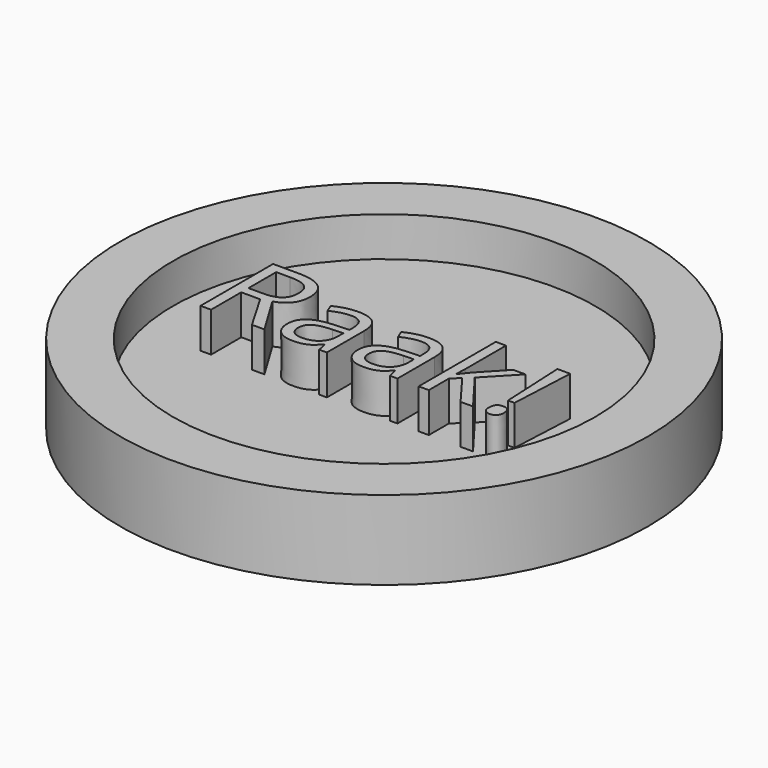
from build123d import *

# Parameters (mm, degrees)
F0_R         = 10
F0_R_2       = 8
F0_TEXT_SIZE = 4.8089487892
F1_DEPTH     = 3
F2_DEPTH     = 1.5


# Not quite as in the source:
# - Text() gives the source's letters only with a copy of the font that has no kerning and outlines rounded to 1/6400 em; it was checked with that copy


with BuildPart() as f1:
    # F0 (on Top) → F1 (new body)
    with BuildSketch(Plane.XY):
        with Locations((-7.6372292832, -17.8669122979)):
            Circle(F0_R)
        with Locations((-7.6372292832, -17.8669122979)):
            Circle(F0_R_2, mode=Mode.SUBTRACT)
        with Locations((-13.6769684032, -19.598133862)):
            Text('Raak!', F0_TEXT_SIZE, font='Open Sans', text_align=(TextAlign.LEFT, TextAlign.BOTTOM))
    extrude(amount=F1_DEPTH)

    # F0 (on Top) → F2 (join)
    with BuildSketch(Plane.XY):
        with Locations((-7.6372292832, -17.8669122979)):
            Circle(F0_R_2)
        with BuildLine():
            Line((-12.0892639045, -18.1704771902), (-12.8060978334, -18.1704771902))
            Line((-12.8060978334, -18.1704771902), (-12.8060978334, -19.598133862))
            Line((-12.8060978334, -19.598133862), (-13.2050903032, -19.598133862))
            Line((-13.2050903032, -19.598133862), (-13.2050903032, -16.1649952655))
            Line((-13.2050903032, -16.1649952655), (-12.2635882981, -16.1649952655))
            add(Edge.make_bspline(
                [(-12.2635882981, -16.1649952655), (-11.6316623713, -16.1649952655), (-11.3299759746, -16.4069455014)],
                knots=[0, 0, 0, 1, 1, 1], degree=2))
            add(Edge.make_bspline(
                [(-11.3299759746, -16.4069455014), (-11.0282895779, -16.6488957374), (-11.0282895779, -17.135050404)],
                knots=[0, 0, 0, 1, 1, 1], degree=2))
            add(Edge.make_bspline(
                [(-11.0282895779, -17.135050404), (-11.0282895779, -17.815817217), (-11.7188245681, -18.0555132582)],
                knots=[0, 0, 0, 1, 1, 1], degree=2))
            Line((-11.7188245681, -18.0555132582), (-10.7863393419, -19.598133862))
            Line((-10.7863393419, -19.598133862), (-11.2582174418, -19.598133862))
            Line((-11.2582174418, -19.598133862), (-12.0892639045, -18.1704771902))
        make_face(mode=Mode.SUBTRACT)
        with BuildLine():
            Line((-8.4194348597, -19.598133862), (-8.7087231853, -19.598133862))
            Line((-8.7087231853, -19.598133862), (-8.7861172049, -19.2314515168))
            Line((-8.7861172049, -19.2314515168), (-8.8049021611, -19.2314515168))
            add(Edge.make_bspline(
                [(-8.8049021611, -19.2314515168), (-8.9972601127, -19.4734017528), (-9.1884909669, -19.5594368522)],
                knots=[0, 0, 0, 1, 1, 1], degree=2))
            add(Edge.make_bspline(
                [(-9.1884909669, -19.5594368522), (-9.3797218211, -19.6454719517), (-9.6667559519, -19.6454719517)],
                knots=[0, 0, 0, 1, 1, 1], degree=2))
            add(Edge.make_bspline(
                [(-9.6667559519, -19.6454719517), (-10.0492176603, -19.6454719517), (-10.2663717541, -19.4478542124)],
                knots=[0, 0, 0, 1, 1, 1], degree=2))
            add(Edge.make_bspline(
                [(-10.2663717541, -19.4478542124), (-10.4835258478, -19.250236473), (-10.4835258478, -18.8865597209)],
                knots=[0, 0, 0, 1, 1, 1], degree=2))
            add(Edge.make_bspline(
                [(-10.4835258478, -18.8865597209), (-10.4835258478, -18.1073597374), (-9.2369561539, -18.0697898249)],
                knots=[0, 0, 0, 1, 1, 1], degree=2))
            Line((-9.2369561539, -18.0697898249), (-8.8003937716, -18.0555132582))
            Line((-8.8003937716, -18.0555132582), (-8.8003937716, -17.8954654313))
            add(Edge.make_bspline(
                [(-8.8003937716, -17.8954654313), (-8.8003937716, -17.5926519373), (-8.9303856686, -17.4483834736)],
                knots=[0, 0, 0, 1, 1, 1], degree=2))
            add(Edge.make_bspline(
                [(-8.9303856686, -17.4483834736), (-9.0603775655, -17.3041150099), (-9.3474116964, -17.3041150099)],
                knots=[0, 0, 0, 1, 1, 1], degree=2))
            add(Edge.make_bspline(
                [(-9.3474116964, -17.3041150099), (-9.6690101467, -17.3041150099), (-10.0747652007, -17.500981351)],
                knots=[0, 0, 0, 1, 1, 1], degree=2))
            Line((-10.0747652007, -17.500981351), (-10.1949889205, -17.2026762464))
            add(Edge.make_bspline(
                [(-10.1949889205, -17.2026762464), (-10.0048851637, -17.0997346864), (-9.7783385918, -17.041125623)],
                knots=[0, 0, 0, 1, 1, 1], degree=2))
            add(Edge.make_bspline(
                [(-9.7783385918, -17.041125623), (-9.5517920199, -16.9825165596), (-9.3233669524, -16.9825165596)],
                knots=[0, 0, 0, 1, 1, 1], degree=2))
            add(Edge.make_bspline(
                [(-9.3233669524, -16.9825165596), (-8.8635112245, -16.9825165596), (-8.6414730421, -17.1865211841)],
                knots=[0, 0, 0, 1, 1, 1], degree=2))
            add(Edge.make_bspline(
                [(-8.6414730421, -17.1865211841), (-8.4194348597, -17.3905258085), (-8.4194348597, -17.8413647575)],
                knots=[0, 0, 0, 1, 1, 1], degree=2))
            Line((-8.4194348597, -17.8413647575), (-8.4194348597, -19.598133862))
        make_face(mode=Mode.SUBTRACT)
        with BuildLine():
            Line((-5.745208494, -19.598133862), (-6.0344968196, -19.598133862))
            Line((-6.0344968196, -19.598133862), (-6.1118908391, -19.2314515168))
            Line((-6.1118908391, -19.2314515168), (-6.1306757953, -19.2314515168))
            add(Edge.make_bspline(
                [(-6.1306757953, -19.2314515168), (-6.3230337469, -19.4734017528), (-6.5142646011, -19.5594368522)],
                knots=[0, 0, 0, 1, 1, 1], degree=2))
            add(Edge.make_bspline(
                [(-6.5142646011, -19.5594368522), (-6.7054954553, -19.6454719517), (-6.9925295862, -19.6454719517)],
                knots=[0, 0, 0, 1, 1, 1], degree=2))
            add(Edge.make_bspline(
                [(-6.9925295862, -19.6454719517), (-7.3749912946, -19.6454719517), (-7.5921453883, -19.4478542124)],
                knots=[0, 0, 0, 1, 1, 1], degree=2))
            add(Edge.make_bspline(
                [(-7.5921453883, -19.4478542124), (-7.8092994821, -19.250236473), (-7.8092994821, -18.8865597209)],
                knots=[0, 0, 0, 1, 1, 1], degree=2))
            add(Edge.make_bspline(
                [(-7.8092994821, -18.8865597209), (-7.8092994821, -18.1073597374), (-6.5627297881, -18.0697898249)],
                knots=[0, 0, 0, 1, 1, 1], degree=2))
            Line((-6.5627297881, -18.0697898249), (-6.1261674059, -18.0555132582))
            Line((-6.1261674059, -18.0555132582), (-6.1261674059, -17.8954654313))
            add(Edge.make_bspline(
                [(-6.1261674059, -17.8954654313), (-6.1261674059, -17.5926519373), (-6.2561593028, -17.4483834736)],
                knots=[0, 0, 0, 1, 1, 1], degree=2))
            add(Edge.make_bspline(
                [(-6.2561593028, -17.4483834736), (-6.3861511998, -17.3041150099), (-6.6731853306, -17.3041150099)],
                knots=[0, 0, 0, 1, 1, 1], degree=2))
            add(Edge.make_bspline(
                [(-6.6731853306, -17.3041150099), (-6.9947837809, -17.3041150099), (-7.400538835, -17.500981351)],
                knots=[0, 0, 0, 1, 1, 1], degree=2))
            Line((-7.400538835, -17.500981351), (-7.5207625547, -17.2026762464))
            add(Edge.make_bspline(
                [(-7.5207625547, -17.2026762464), (-7.3306587979, -17.0997346864), (-7.104112226, -17.041125623)],
                knots=[0, 0, 0, 1, 1, 1], degree=2))
            add(Edge.make_bspline(
                [(-7.104112226, -17.041125623), (-6.8775656542, -16.9825165596), (-6.6491405867, -16.9825165596)],
                knots=[0, 0, 0, 1, 1, 1], degree=2))
            add(Edge.make_bspline(
                [(-6.6491405867, -16.9825165596), (-6.1892848587, -16.9825165596), (-5.9672466763, -17.1865211841)],
                knots=[0, 0, 0, 1, 1, 1], degree=2))
            add(Edge.make_bspline(
                [(-5.9672466763, -17.1865211841), (-5.745208494, -17.3905258085), (-5.745208494, -17.8413647575)],
                knots=[0, 0, 0, 1, 1, 1], degree=2))
            Line((-5.745208494, -17.8413647575), (-5.745208494, -19.598133862))
        make_face(mode=Mode.SUBTRACT)
        with BuildLine():
            add(Edge.make_bspline(
                [(-2.3950994039, -19.5924983752), (-2.4751233173, -19.5184856477), (-2.4751233173, -19.3494210418)],
                knots=[0, 0, 0, 1, 1, 1], degree=2))
            add(Edge.make_bspline(
                [(-2.4751233173, -19.3494210418), (-2.4751233173, -19.0300767863), (-2.1933489742, -19.0300767863)],
                knots=[0, 0, 0, 1, 1, 1], degree=2))
            add(Edge.make_bspline(
                [(-2.1933489742, -19.0300767863), (-2.0573458912, -19.0300767863), (-1.9833331638, -19.1119791954)],
                knots=[0, 0, 0, 1, 1, 1], degree=2))
            add(Edge.make_bspline(
                [(-1.9833331638, -19.1119791954), (-1.9093204363, -19.1938816044), (-1.9093204363, -19.3494210418)],
                knots=[0, 0, 0, 1, 1, 1], degree=2))
            add(Edge.make_bspline(
                [(-1.9093204363, -19.3494210418), (-1.9093204363, -19.4997006915), (-1.9844602612, -19.5831058971)],
                knots=[0, 0, 0, 1, 1, 1], degree=2))
            add(Edge.make_bspline(
                [(-1.9844602612, -19.5831058971), (-2.059600086, -19.6665111026), (-2.1933489742, -19.6665111026)],
                knots=[0, 0, 0, 1, 1, 1], degree=2))
            add(Edge.make_bspline(
                [(-2.1933489742, -19.6665111026), (-2.3150754904, -19.6665111026), (-2.3950994039, -19.5924983752)],
                knots=[0, 0, 0, 1, 1, 1], degree=2))
        make_face(mode=Mode.SUBTRACT)
        with BuildLine():
            Line((-4.5760328196, -18.2809327327), (-4.5572478634, -18.2809327327))
            add(Edge.make_bspline(
                [(-4.5572478634, -18.2809327327), (-4.4565604981, -18.1374156673), (-4.2499259798, -17.9052336086)],
                knots=[0, 0, 0, 1, 1, 1], degree=2))
            Line((-4.2499259798, -17.9052336086), (-3.4188795172, -17.0245948615))
            Line((-3.4188795172, -17.0245948615), (-2.9560181962, -17.0245948615))
            Line((-2.9560181962, -17.0245948615), (-3.9989589649, -18.1208849058))
            Line((-3.9989589649, -18.1208849058), (-2.8831325661, -19.598133862))
            Line((-2.8831325661, -19.598133862), (-3.3550106661, -19.598133862))
            Line((-3.3550106661, -19.598133862), (-4.2642025465, -18.381620098))
            Line((-4.2642025465, -18.381620098), (-4.5572478634, -18.6355927059))
            Line((-4.5572478634, -18.6355927059), (-4.5572478634, -19.598133862))
            Line((-4.5572478634, -19.598133862), (-4.9427151648, -19.598133862))
            Line((-4.9427151648, -19.598133862), (-4.9427151648, -15.9440841805))
            Line((-4.9427151648, -15.9440841805), (-4.5572478634, -15.9440841805))
            Line((-4.5572478634, -15.9440841805), (-4.5572478634, -17.8819402629))
            add(Edge.make_bspline(
                [(-4.5572478634, -17.8819402629), (-4.5572478634, -18.0104293633), (-4.5760328196, -18.2809327327)],
                knots=[0, 0, 0, 1, 1, 1], degree=2))
        make_face(mode=Mode.SUBTRACT)
        Polygon((-1.9468903487, -16.1649952655), (-2.0663626702, -18.6521234674), (-2.3128212957, -18.6521234674), (-2.4330450154, -16.1649952655), align=None, mode=Mode.SUBTRACT)
        with BuildLine():
            Line((-12.8060978334, -16.5151468492), (-12.8060978334, -17.827839589))
            Line((-12.8060978334, -17.827839589), (-12.2583285103, -17.827839589))
            add(Edge.make_bspline(
                [(-12.2583285103, -17.827839589), (-11.8360426948, -17.827839589), (-11.6388006546, -17.6599020805)],
                knots=[0, 0, 0, 1, 1, 1], degree=2))
            add(Edge.make_bspline(
                [(-11.6388006546, -17.6599020805), (-11.4415586144, -17.491964572), (-11.4415586144, -17.156089555)],
                knots=[0, 0, 0, 1, 1, 1], degree=2))
            add(Edge.make_bspline(
                [(-11.4415586144, -17.156089555), (-11.4415586144, -16.8157061485), (-11.6421819467, -16.6654264989)],
                knots=[0, 0, 0, 1, 1, 1], degree=2))
            add(Edge.make_bspline(
                [(-11.6421819467, -16.6654264989), (-11.842805279, -16.5151468492), (-12.2868816438, -16.5151468492)],
                knots=[0, 0, 0, 1, 1, 1], degree=2))
            Line((-12.2868816438, -16.5151468492), (-12.8060978334, -16.5151468492))
        make_face()
        with BuildLine():
            add(Edge.make_bspline(
                [(-9.9470274985, -19.2130422598), (-9.8192897963, -19.3231221031), (-9.5893619323, -19.3231221031)],
                knots=[0, 0, 0, 1, 1, 1], degree=2))
            add(Edge.make_bspline(
                [(-9.5893619323, -19.3231221031), (-9.2249337819, -19.3231221031), (-9.0171721662, -19.1236258682)],
                knots=[0, 0, 0, 1, 1, 1], degree=2))
            add(Edge.make_bspline(
                [(-9.0171721662, -19.1236258682), (-8.8094105506, -18.9241296333), (-8.8094105506, -18.5649612706)],
                knots=[0, 0, 0, 1, 1, 1], degree=2))
            Line((-8.8094105506, -18.5649612706), (-8.8094105506, -18.3327792119))
            Line((-8.8094105506, -18.3327792119), (-9.1993862415, -18.3485585751))
            add(Edge.make_bspline(
                [(-9.1993862415, -18.3485585751), (-9.6645017572, -18.3650893365), (-9.869633479, -18.4932027379)],
                knots=[0, 0, 0, 1, 1, 1], degree=2))
            add(Edge.make_bspline(
                [(-9.869633479, -18.4932027379), (-10.0747652007, -18.6213161392), (-10.0747652007, -18.8910681104)],
                knots=[0, 0, 0, 1, 1, 1], degree=2))
            add(Edge.make_bspline(
                [(-10.0747652007, -18.8910681104), (-10.0747652007, -19.1029624164), (-9.9470274985, -19.2130422598)],
                knots=[0, 0, 0, 1, 1, 1], degree=2))
        make_face()
        with BuildLine():
            add(Edge.make_bspline(
                [(-7.2728011328, -19.2130422598), (-7.1450634306, -19.3231221031), (-6.9151355666, -19.3231221031)],
                knots=[0, 0, 0, 1, 1, 1], degree=2))
            add(Edge.make_bspline(
                [(-6.9151355666, -19.3231221031), (-6.5507074162, -19.3231221031), (-6.3429458005, -19.1236258682)],
                knots=[0, 0, 0, 1, 1, 1], degree=2))
            add(Edge.make_bspline(
                [(-6.3429458005, -19.1236258682), (-6.1351841848, -18.9241296333), (-6.1351841848, -18.5649612706)],
                knots=[0, 0, 0, 1, 1, 1], degree=2))
            Line((-6.1351841848, -18.5649612706), (-6.1351841848, -18.3327792119))
            Line((-6.1351841848, -18.3327792119), (-6.5251598757, -18.3485585751))
            add(Edge.make_bspline(
                [(-6.5251598757, -18.3485585751), (-6.9902753914, -18.3650893365), (-7.1954071132, -18.4932027379)],
                knots=[0, 0, 0, 1, 1, 1], degree=2))
            add(Edge.make_bspline(
                [(-7.1954071132, -18.4932027379), (-7.400538835, -18.6213161392), (-7.400538835, -18.8910681104)],
                knots=[0, 0, 0, 1, 1, 1], degree=2))
            add(Edge.make_bspline(
                [(-7.400538835, -18.8910681104), (-7.400538835, -19.1029624164), (-7.2728011328, -19.2130422598)],
                knots=[0, 0, 0, 1, 1, 1], degree=2))
        make_face()
    extrude(amount=F2_DEPTH)


solid = f1.part
